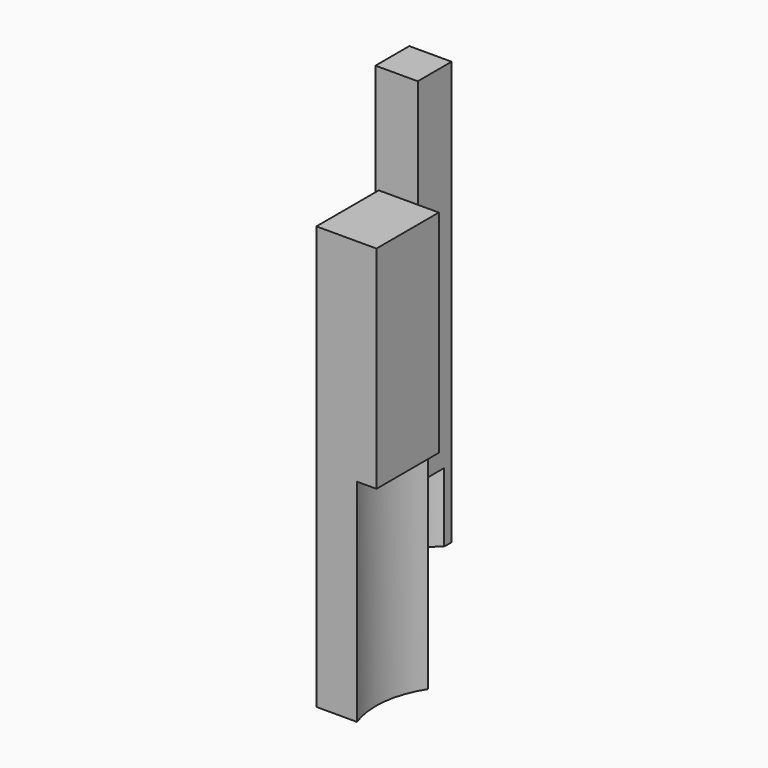
from build123d import *

# Parameters (mm, degrees)
F1_W     = 50.8
F1_H     = 50.8
F2_DEPTH = 508
F3_R     = 63.5
F4_DEPTH = 83.05869
F5_W     = 72.1005052328
F5_H     = 93.6214327812
F6_DEPTH = 508
F7_R     = 105.920672741
F8_DEPTH = 254


# Not quite as in the source:
# - a variable given as a bare number and used for a length is read in inches; the dataset says mm whatever the document's units were


with BuildPart() as f2:
    # F1 (on Top) → F2 (new body)
    with BuildSketch(Plane.XY):
        with Locations((9.6655465204, -15.6340606053)):
            Rectangle(F1_W, F1_H)
    extrude(amount=F2_DEPTH)

    # F3 (on Top) → F4 (cut)
    with BuildSketch(Plane.XY):
        with Locations((72.4574252963, -52.7999475598)):
            Circle(F3_R)
    extrude(amount=F4_DEPTH, mode=Mode.SUBTRACT)


with BuildPart() as f6:
    # F5 (on Top) → F6 (new body)
    with BuildSketch(Plane.XY):
        with Locations((180.9576675296, -283.6835384369)):
            Rectangle(F5_W, F5_H)
    extrude(amount=F6_DEPTH)

    # F7 (on Top) → F8 (cut)
    with BuildSketch(Plane.XY):
        with Locations((293.1186258793, -294.1574752331)):
            Circle(F7_R)
    extrude(amount=F8_DEPTH, mode=Mode.SUBTRACT)


solid = Compound([f2.part, f6.part])
